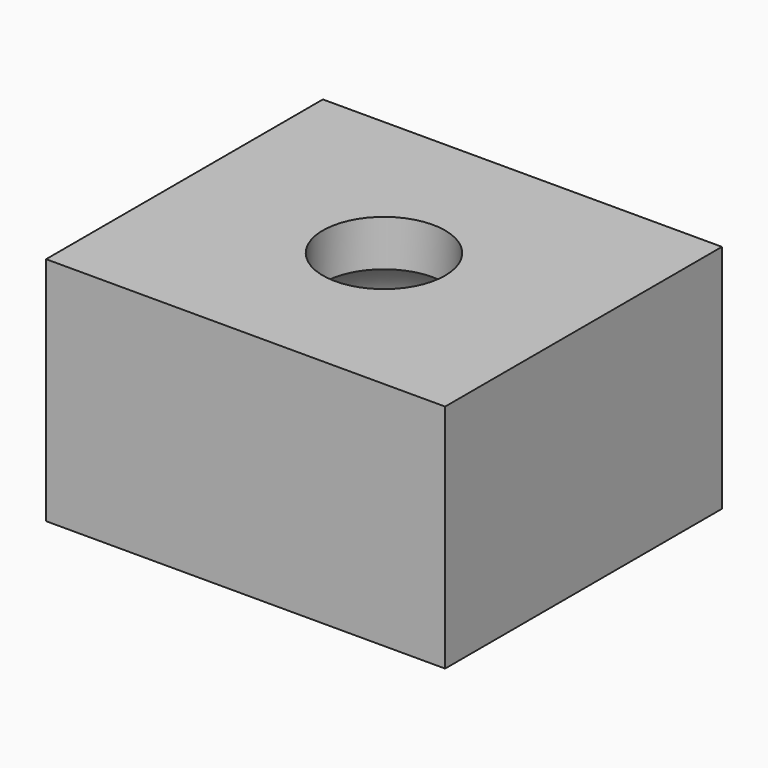
from build123d import *

# Parameters (mm, degrees)
F0_W     = 17.3
F0_H     = 15
F0_R     = 5.65
F1_DEPTH = 10
F2_DEPTH = 8
F3_R     = 2.65
F4_DEPTH = 16.1


# Not quite as in the source:
# - a fillet or chamfer that OpenCascade refuses, or shapes differently, is made with other operations: its cross-section is extruded or revolved along the edge and cut away or added


with BuildPart() as f1:
    # F0 (on Top) → F1 (new body)
    with BuildSketch(Plane.XY):
        Rectangle(F0_W, F0_H)
        Circle(F0_R, mode=Mode.SUBTRACT)
        Circle(F0_R)
    extrude(amount=F1_DEPTH)

    # F0 (on Top) → F2 (cut)
    with BuildSketch(Plane.XY):
        Circle(F0_R)
    extrude(amount=F2_DEPTH, mode=Mode.SUBTRACT)

    # F3 (on face) → F4 (cut)
    with BuildSketch(Plane.XY):
        Circle(F3_R)
    extrude(amount=F4_DEPTH, mode=Mode.SUBTRACT)

    # F5: fillet of radius 4 on 1 edges, made by hand

    # F5_s1 → F5_t2 (revolve)
    with BuildSketch(Plane.XZ):
        with BuildLine():
            ThreePointArc((5.65, 4.1270166538), (4.8122776602, 6.5765063966), (2.65, 8))
            Line((2.65, 8), (5.65, 8))
            Line((5.65, 8), (5.65, 4.1270166538))
        make_face()
    revolve(axis=Axis((0, 0, 8), (0, 0, 1)))


solid = f1.part
